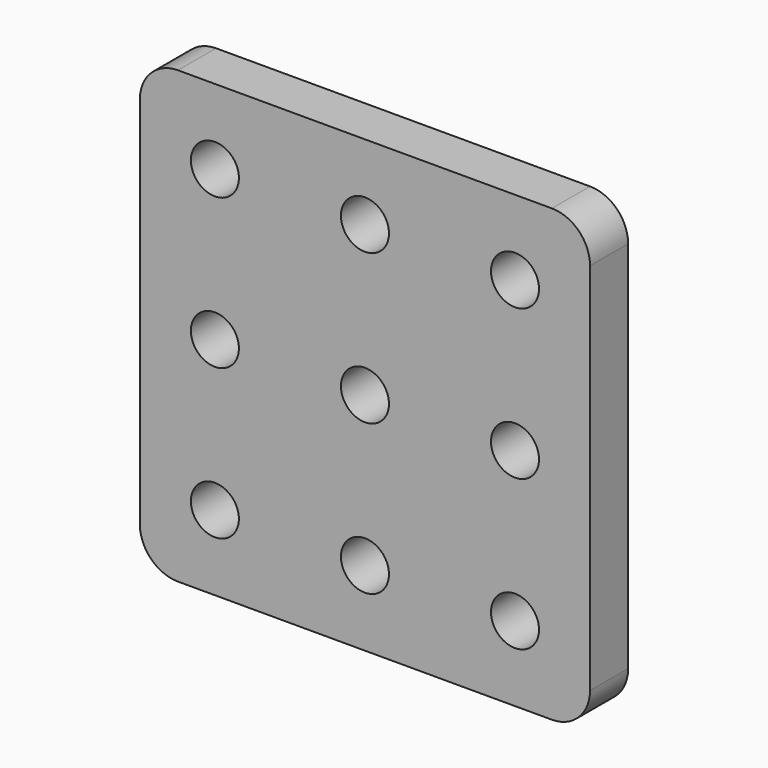
from build123d import *

# Parameters (mm, degrees)
F0_R     = 1.6
F1_DEPTH = 3.175


# Not quite as in the source:
# - a length typed as a fraction of an inch, garbled in the dataset ("3 / 203.2 mm" for 3/8 in), is restored


with BuildPart() as f1:
    # F0 (on Front) → F1 (new body)
    with BuildSketch(Plane.XZ):
        with BuildLine():
            Line((27.46, 0), (2.54, 0))
            ThreePointArc((2.54, 0), (0.7439487758, -0.7439487758), (0, -2.54))
            Line((0, -2.54), (0, -27.46))
            ThreePointArc((0, -27.46), (0.7439487758, -29.2560512242), (2.54, -30))
            Line((2.54, -30), (27.46, -30))
            ThreePointArc((27.46, -30), (29.2560512242, -29.2560512242), (30, -27.46))
            Line((30, -27.46), (30, -2.54))
            ThreePointArc((30, -2.54), (29.2560512242, -0.7439487758), (27.46, 0))
        make_face()
        with Locations((5, -25)):
            Circle(F0_R, mode=Mode.SUBTRACT)
        with Locations((15, -25)):
            Circle(F0_R, mode=Mode.SUBTRACT)
        with Locations((25, -25)):
            Circle(F0_R, mode=Mode.SUBTRACT)
        with Locations((5, -15)):
            Circle(F0_R, mode=Mode.SUBTRACT)
        with Locations((5, -5)):
            Circle(F0_R, mode=Mode.SUBTRACT)
        with Locations((15, -15)):
            Circle(F0_R, mode=Mode.SUBTRACT)
        with Locations((25, -15)):
            Circle(F0_R, mode=Mode.SUBTRACT)
        with Locations((15, -5)):
            Circle(F0_R, mode=Mode.SUBTRACT)
        with Locations((25, -5)):
            Circle(F0_R, mode=Mode.SUBTRACT)
    extrude(amount=F1_DEPTH)


solid = f1.part
